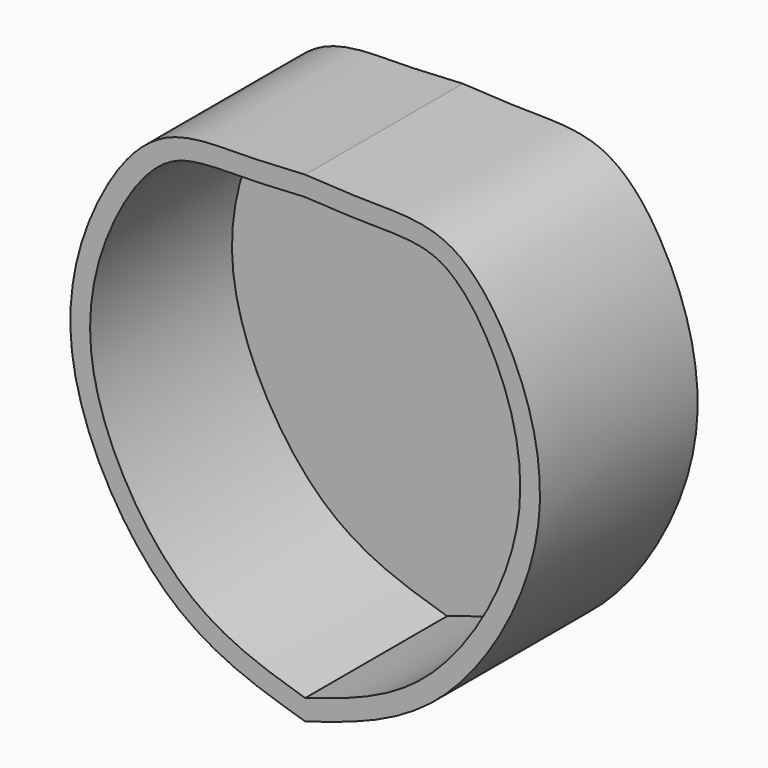
from build123d import *

# Parameters (mm, degrees)
F1_DEPTH = 25
F2_T     = -2.5


with BuildPart() as f1:
    # F0 (on Front) → F1 (new body)
    with BuildSketch(Plane.XZ):
        with BuildLine():
            add(Edge.make_bspline(
                [(0, 61.0584691167), (2.7496223119, 60.8971283441), (8.3909718756, 60.5661084463), (18.5972333394, 60.849734506), (27.1211390751, 50.2998999845), (32.7609921647, 30.4950267283), (18.6978379575, 5.64333428), (5.8838131464, 1.7758376397), (0, 0)],
                knots=[0, 0, 0, 0, 0.124507946, 0.2554506645, 0.4051343765, 0.5955446281, 0.8142863098, 1, 1, 1, 1], degree=3))
            add(Edge.make_bspline(
                [(0, 61.0584691167), (-2.7496223119, 60.8971283441), (-8.3909718756, 60.5661084463), (-18.5972333394, 60.849734506), (-27.1211390751, 50.2998999845), (-32.7609921647, 30.4950267283), (-18.6978379575, 5.64333428), (-5.8838131464, 1.7758376397), (0, 0)],
                knots=[0, 0, 0, 0, 0.124507946, 0.2554506645, 0.4051343765, 0.5955446281, 0.8142863098, 1, 1, 1, 1], degree=3))
        make_face()
    extrude(amount=F1_DEPTH)

    # F2
    f2_openings = [f1.faces().sort_by_distance(p)[0] for p in [
        (0, -25, 32.818445),
    ]]
    offset(amount=F2_T, openings=f2_openings)


solid = f1.part
